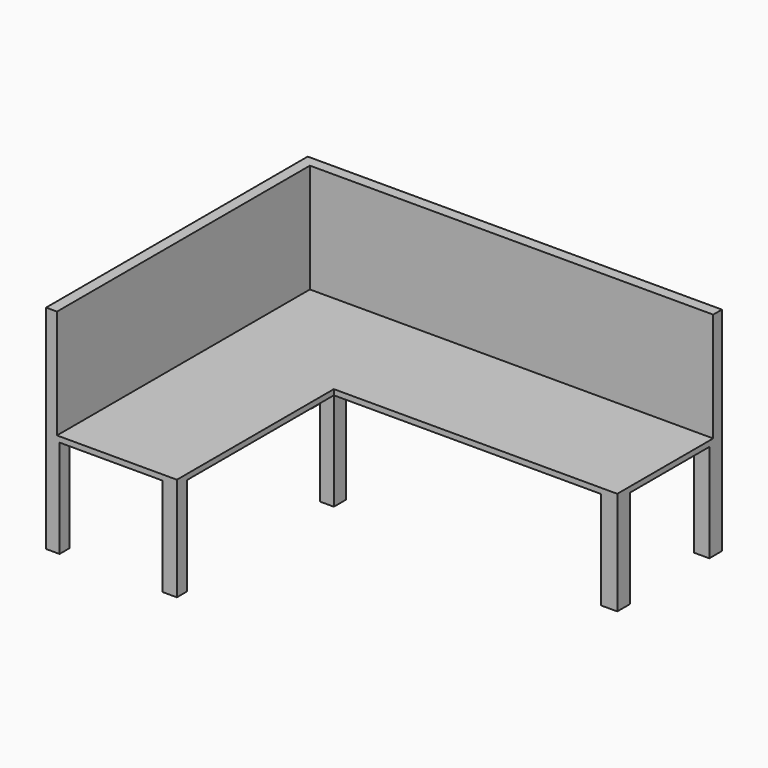
from build123d import *

# Parameters (mm, degrees)
F1_DEPTH = 25
F3_DEPTH = 500
F4_W     = 61.7009438574
F4_H     = 57.8163862228
F4_W_2   = 65.7990336418
F4_W_3   = 62.8085494041
F4_H_2   = 69.920873642
F4_H_3   = 57.5791224837
F4_W_4   = 73.9003658295
F4_H_4   = 72.9114174843
F4_W_5   = 70.9098815918
F4_H_5   = 72.5316330791
F5_DEPTH = 450


with BuildPart() as f1:
    # F0 (on Top) → F1 (new body)
    with BuildSketch(Plane.XY):
        Polygon((1900, 0), (0, 0), (0, -600), (0, -1500), (600, -1500), (600, -600), (1900, -600), align=None)
    extrude(amount=F1_DEPTH)

    # F2 (on face) → F3 (join)
    with BuildSketch(Plane.XY.offset(25)):
        Polygon((1900, -50), (1900, 0), (0, 0), (0, -50), (0, -231.5181791782), (0, -1500), (50, -1500), (50, -50), align=None)
    extrude(amount=F3_DEPTH)

    # F4 (on face) → F5 (join)
    with BuildSketch(Plane(origin=(0, 0, 0), x_dir=(1, 0, 0), z_dir=(0, 0, -1))):
        with Locations((30.8504719287, 1471.0918068886)):
            Rectangle(F4_W, F4_H)
        with Locations((567.1004831791, 1471.0918068886)):
            Rectangle(F4_W_2, F4_H)
        with Locations((568.5957252979, 565.039563179)):
            Rectangle(F4_W_3, F4_H_2)
        with Locations((30.8504719287, 28.7895612419)):
            Rectangle(F4_W, F4_H_3)
        with Locations((1863.0498170853, 563.5442912579)):
            Rectangle(F4_W_4, F4_H_4)
        with Locations((1864.5450592041, 36.2658165395)):
            Rectangle(F4_W_5, F4_H_5)
    extrude(amount=F5_DEPTH)


solid = f1.part
